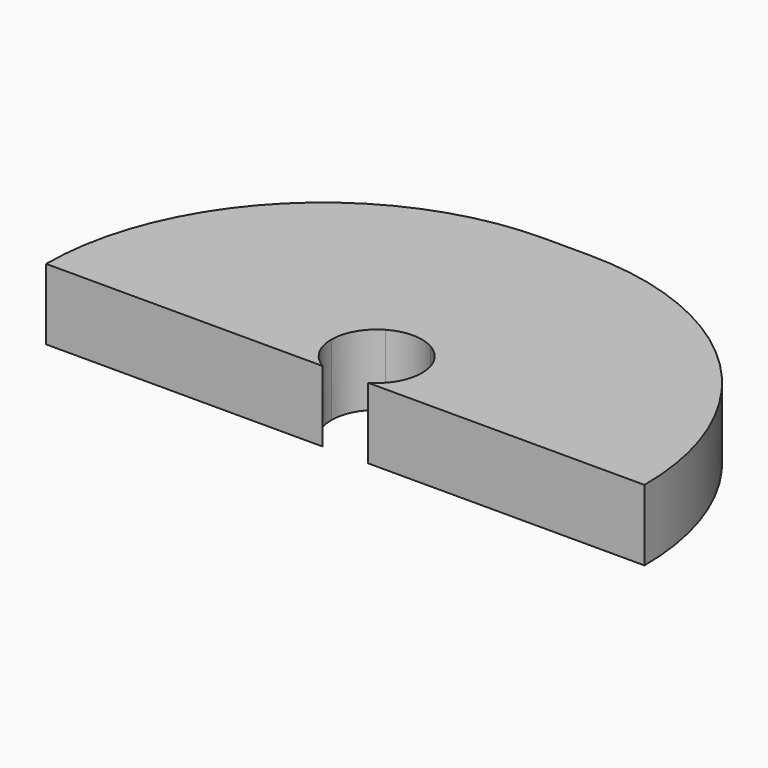
from build123d import *

# Parameters (mm, degrees)
F1_DEPTH = 5


with BuildPart() as f1:
    # F0 (on Top) → F1 (new body)
    with BuildSketch(Plane.XY):
        with BuildLine():
            ThreePointArc((3.1956666573, -6.9824714928), (2.7675285072, -8.5803048214), (1.5978333287, -9.75))
            Line((1.5978333287, -9.75), (4.793499986, -9.75))
            ThreePointArc((4.793499986, -9.75), (4.3653618359, -8.1521666713), (3.1956666573, -6.9824714928))
        make_face()
        with BuildLine():
            Line((-4.793499986, -9.75), (-1.5978333286, -9.75))
            ThreePointArc((-1.5978333286, -9.75), (-2.7675285072, -8.5803048214), (-3.1956666573, -6.9824714928))
            ThreePointArc((-3.1956666573, -6.9824714928), (-4.3653618359, -8.1521666713), (-4.793499986, -9.75))
        make_face()
        with BuildLine():
            ThreePointArc((3.1956666573, -6.9824714928), (4.3653618359, -8.1521666713), (4.793499986, -9.75))
            Line((4.793499986, -9.75), (12.3826613305, -9.75))
            Line((12.3826613305, -9.75), (17.9021666714, -9.75))
            ThreePointArc((17.9021666714, -9.75), (13.2777422874, 2.8582215277), (1.5978333286, 9.4863643814))
            Line((1.5978333286, 9.4863643814), (1.5978333287, -4.2149429855))
            ThreePointArc((1.5978333286, -4.2149429855), (2.7675285072, -5.3846381641), (3.1956666573, -6.9824714928))
        make_face()
        with BuildLine():
            Line((-17.9021666713, -9.75), (-4.793499986, -9.75))
            ThreePointArc((-4.793499986, -9.75), (-4.3653618359, -8.1521666713), (-3.1956666573, -6.9824714928))
            ThreePointArc((-3.1956666573, -6.9824714928), (-2.7675285072, -5.3846381641), (-1.5978333287, -4.2149429855))
            Line((-1.5978333286, -4.2149429855), (-1.5978333287, 9.4863643814))
            ThreePointArc((-1.5978333287, 9.4863643814), (-13.2777422874, 2.8582215277), (-17.9021666713, -9.75))
        make_face()
        with BuildLine():
            ThreePointArc((-1.5978333287, -4.2149429855), (0, -3.7868048355), (1.5978333286, -4.2149429855))
            Line((1.5978333287, -4.2149429855), (1.5978333286, 9.4863643814))
            ThreePointArc((1.5978333286, 9.4863643814), (0.8009617163, 9.6018935077), (0, 9.6844263783))
            ThreePointArc((0, 9.6844263783), (-0.8009617163, 9.6018935077), (-1.5978333287, 9.4863643814))
            Line((-1.5978333287, 9.4863643814), (-1.5978333286, -4.2149429855))
        make_face()
        with BuildLine():
            Line((-21.0978333287, -9.75), (-17.9021666713, -9.75))
            ThreePointArc((-17.9021666713, -9.75), (-13.2777422874, 2.8582215277), (-1.5978333287, 9.4863643814))
            Line((-1.5978333287, 9.4863643814), (-1.5978333287, 9.75))
            ThreePointArc((-1.5978333287, 9.75), (-15.3864155618, 4.0385822331), (-21.0978333286, -9.75))
        make_face()
        with BuildLine():
            ThreePointArc((0, 9.6844263783), (0.8009617163, 9.6018935077), (1.5978333286, 9.4863643814))
            Line((1.5978333286, 9.4863643814), (1.5978333286, 9.75))
            ThreePointArc((1.5978333286, 9.75), (0.798244177, 9.7335996979), (0, 9.6844263783))
        make_face()
        with BuildLine():
            Line((1.5978333286, 9.75), (1.5978333286, 9.4863643814))
            ThreePointArc((1.5978333286, 9.4863643814), (13.2777422874, 2.8582215277), (17.9021666714, -9.75))
            Line((17.9021666714, -9.75), (21.0978333287, -9.75))
            ThreePointArc((21.0978333287, -9.75), (15.3864155618, 4.0385822331), (1.5978333286, 9.75))
        make_face()
        with BuildLine():
            Line((-1.5978333287, 9.75), (-1.5978333287, 9.4863643814))
            ThreePointArc((-1.5978333287, 9.4863643814), (-0.8009617163, 9.6018935077), (0, 9.6844263783))
            ThreePointArc((0, 9.6844263783), (-0.798244177, 9.7335996979), (-1.5978333287, 9.75))
        make_face()
        with BuildLine():
            ThreePointArc((0, 9.6844263783), (0.798244177, 9.7335996979), (1.5978333286, 9.75))
            Line((1.5978333286, 9.75), (-1.5978333287, 9.75))
            ThreePointArc((-1.5978333287, 9.75), (-0.798244177, 9.7335996979), (0, 9.6844263783))
        make_face()
    extrude(amount=F1_DEPTH)


solid = f1.part
